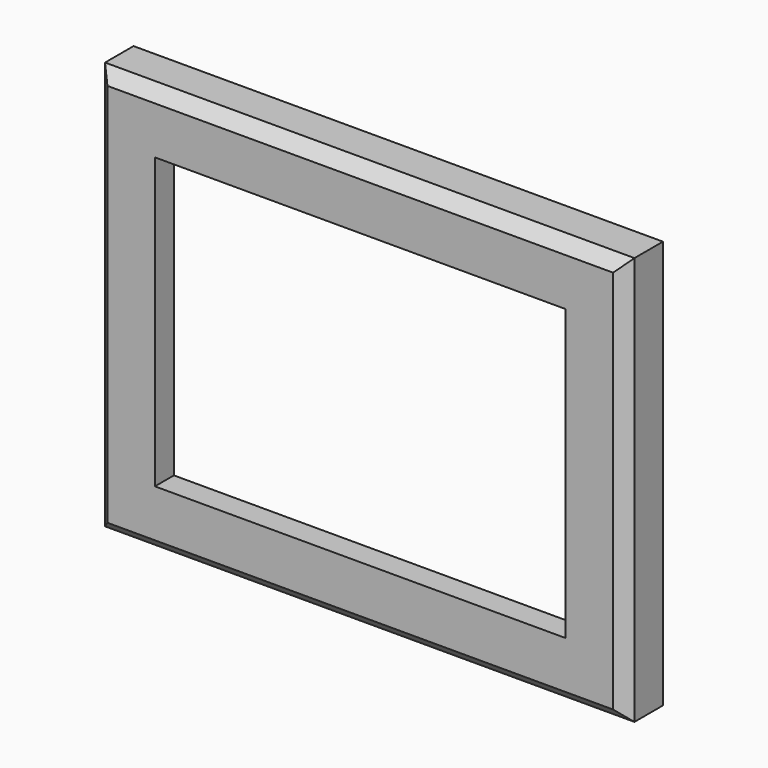
from build123d import *

# Parameters (mm, degrees)
F0_W     = 223
F0_H     = 172
F0_W_2   = 189
F0_H_2   = 138
F0_W_3   = 173
F0_H_3   = 122
F1_DEPTH = 20
F2_SIZE  = 5
F3_DEPTH = 10


# Not quite as in the source:
# - a feature names something its author has since deleted; it is built from what else it names


with BuildPart() as f1:
    # F0 (on Front) → F1 (new body)
    with BuildSketch(Plane.XZ):
        Rectangle(F0_W, F0_H)
        Rectangle(F0_W_2, F0_H_2, mode=Mode.SUBTRACT)
        Rectangle(F0_W_2, F0_H_2)
        Rectangle(F0_W_3, F0_H_3, mode=Mode.SUBTRACT)
    extrude(amount=F1_DEPTH)

    # F2
    f2_edges = [f1.edges().sort_by_distance(p)[0] for p in [
        (-111.5, -20, 0),
        (0, -20, 86),
        (111.5, -20, 0),
        (0, -20, -86),
    ]]
    chamfer(f2_edges, length=F2_SIZE)

    # F0 (on Front) → F3 (cut)
    with BuildSketch(Plane.XZ):
        Rectangle(F0_W_2, F0_H_2)
        Rectangle(F0_W_3, F0_H_3, mode=Mode.SUBTRACT)
    extrude(amount=F3_DEPTH, mode=Mode.SUBTRACT)


solid = f1.part
